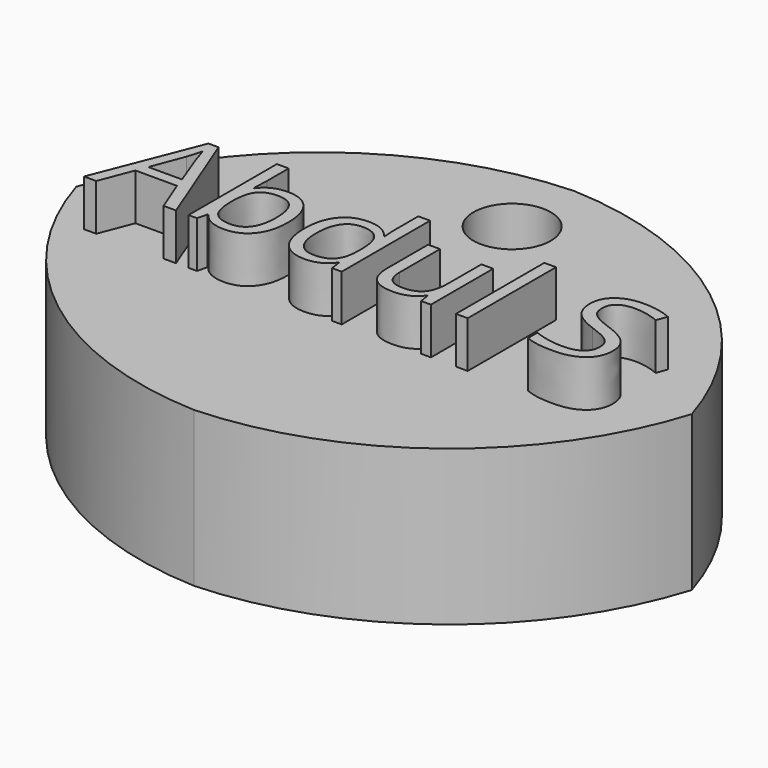
from build123d import *

# Parameters (mm, degrees)
F0_W         = 125
F0_H         = 92.0479061162
F1_DEPTH     = 30
F2_TEXT_SIZE = 28.1628162816
F3_DEPTH     = 9
F5_DEPTH     = 128.6
F6_T1_DEPTH  = 355.9188309204


# Not quite as in the source:
# - a fillet or chamfer that OpenCascade refuses, or shapes differently, is made with other operations: its cross-section is extruded or revolved along the edge and cut away or added
# - Text() gives the source's letters only with a copy of the font that has no kerning and outlines rounded to 1/6400 em; it was checked with that copy


with BuildPart() as f1:
    # F0 (on Top) → F1 (new body)
    with BuildSketch(Plane.XY):
        Rectangle(F0_W, F0_H)
    extrude(amount=F1_DEPTH)

    # F2 (on face) → F3 (join)
    with BuildSketch(Plane.XY.offset(30)):
        with Locations((-50, -10.1386138614)):
            Text('Abdul S', F2_TEXT_SIZE, font='Open Sans', text_align=(TextAlign.LEFT, TextAlign.BOTTOM))
    extrude(amount=F3_DEPTH)

    # F4 (on face) → F5 (cut)
    with BuildSketch(Plane.XY.offset(30)):
        with BuildLine():
            ThreePointArc((0, 38.5239530581), (-5.3033008589, 25.7206521992), (7.5, 31.0239530581))
            ThreePointArc((7.5, 31.0239530581), (5.3033008589, 36.327253917), (0, 38.5239530581))
        make_face()
    extrude(amount=-F5_DEPTH, mode=Mode.SUBTRACT)

    # F6: fillet of radius 65.1837661841 on 4 edges, made by hand

    # F6_s2 → F6_t1 (cut)
    with BuildSketch(Plane.XY.offset(-162.9594154602)):
        with BuildLine():
            ThreePointArc((62.5, -19.159813126), (43.408116908, 26.9320699661), (-2.6837661841, 46.0239530581))
            Line((-2.6837661841, 46.0239530581), (62.5, 46.0239530581))
            Line((62.5, 46.0239530581), (62.5, -19.159813126))
        make_face()
        with BuildLine():
            ThreePointArc((62.5, 19.159813126), (43.408116908, -26.9320699661), (-2.6837661841, -46.0239530581))
            Line((-2.6837661841, -46.0239530581), (62.5, -46.0239530581))
            Line((62.5, -46.0239530581), (62.5, 19.159813126))
        make_face()
        with BuildLine():
            ThreePointArc((2.6837661841, -46.0239530581), (-43.408116908, -26.9320699661), (-62.5, 19.159813126))
            Line((-62.5, 19.159813126), (-62.5, -46.0239530581))
            Line((-62.5, -46.0239530581), (2.6837661841, -46.0239530581))
        make_face()
        with BuildLine():
            ThreePointArc((2.6837661841, 46.0239530581), (-43.408116908, 26.9320699661), (-62.5, -19.159813126))
            Line((-62.5, -19.159813126), (-62.5, 46.0239530581))
            Line((-62.5, 46.0239530581), (2.6837661841, 46.0239530581))
        make_face()
    extrude(amount=F6_T1_DEPTH, mode=Mode.SUBTRACT)


solid = f1.part
